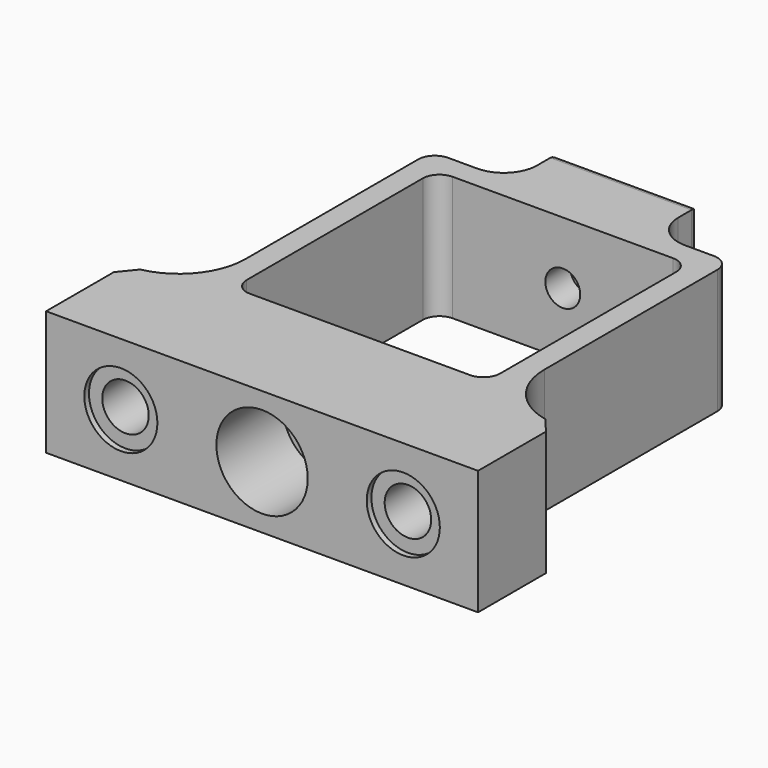
from build123d import *

# Parameters (mm, degrees)
F1_DEPTH       = 15
F2_T1_DEPTH    = 24.3030738828
F4_R           = 5.5
F5_DEPTH       = 6
F6_R           = 1
F7_R           = 2.1
F8_DEPTH       = 3.75
F9_R           = 5.5
F10_DEPTH      = 10
F10_DEPTH_BACK = 25
F11_R          = 2.1
F12_DEPTH      = 14.75
F3_R           = 2.8
F13_DEPTH      = 6.5
F14_R          = 4.4
F15_DEPTH      = 0.7


# Not quite as in the source:
# - a fillet or chamfer that OpenCascade refuses, or shapes differently, is made with other operations: its cross-section is extruded or revolved along the edge and cut away or added


with BuildPart() as f1:
    # F0 (on Top) → F1 (new body)
    with BuildSketch(Plane.XY):
        with BuildLine():
            ThreePointArc((18, 16), (17.4142135624, 17.4142135624), (16, 18))
            Line((16, 18), (12.5, 18))
            ThreePointArc((12.5, 18), (9.6715728753, 19.1715728753), (8.5, 22))
            Line((8.5, 22), (8.5, 25))
            Line((8.5, 25), (-8.5, 25))
            Line((-8.5, 25), (-8.5, 22))
            ThreePointArc((-8.5, 22), (-9.6715728753, 19.1715728753), (-12.5, 18))
            Line((-12.5, 18), (-16, 18))
            ThreePointArc((-16, 18), (-17.4142135624, 17.4142135624), (-18, 16))
            Line((-18, 16), (-18, -10))
            ThreePointArc((-18, -10), (-20.3431457505, -15.6568542495), (-26, -18))
            Line((-26, -18), (-26, -30))
            Line((-26, -30), (26, -30))
            Line((26, -30), (26, -18))
            ThreePointArc((26, -18), (20.3431457505, -15.6568542495), (18, -10))
            Line((18, -10), (18, 16))
        make_face()
        with BuildLine():
            Line((-13.25, 15.25), (13.25, 15.25))
            ThreePointArc((13.25, 15.25), (14.6642135624, 14.6642135624), (15.25, 13.25))
            Line((15.25, 13.25), (15.25, -13.25))
            ThreePointArc((15.25, -13.25), (14.6642135624, -14.6642135624), (13.25, -15.25))
            Line((13.25, -15.25), (-13.25, -15.25))
            ThreePointArc((-13.25, -15.25), (-14.6642135624, -14.6642135624), (-15.25, -13.25))
            Line((-15.25, -13.25), (-15.25, 13.25))
            ThreePointArc((-15.25, 13.25), (-14.6642135624, 14.6642135624), (-13.25, 15.25))
        make_face(mode=Mode.SUBTRACT)
    extrude(amount=F1_DEPTH)

    # F2: chamfer of 2 on 2 edges, made by hand

    # F2_s2 → F2_t1 (cut)
    with BuildSketch(Plane.XY.offset(-4.6515369414)):
        with BuildLine():
            Line((-24.4, -17.8383671769), (-26, -19.7979589711))
            Line((-26, -19.7979589711), (-26, -18))
            ThreePointArc((-26, -18), (-25.1675484588, -17.9565711479), (-24.4, -17.8383671769))
        make_face()
        with BuildLine():
            Line((26, -19.7979589711), (24.4, -17.8383671769))
            ThreePointArc((24.4, -17.8383671769), (25.1675484588, -17.9565711479), (26, -18))
            Line((26, -18), (26, -19.7979589711))
        make_face()
    extrude(amount=F2_T1_DEPTH, mode=Mode.SUBTRACT)

    # F4 (on face) → F5 (cut)
    with BuildSketch(Plane(origin=(0, 25, 0), x_dir=(-1, 0, 0), z_dir=(0, 1, 0))):
        with Locations((0, 7.5)):
            Circle(F4_R)
    extrude(amount=-F5_DEPTH, mode=Mode.SUBTRACT)

    # F6
    f6_edges = [f1.edges().sort_by_distance(p)[0] for p in [
        (0, 25, 0),
        (-8.5, 25, 7.5),
        (0, 25, 15),
        (8.5, 25, 7.5),
    ]]
    fillet(f6_edges, radius=F6_R)

    # F7 (on face) → F8 (cut, through all)
    with BuildSketch(Plane(origin=(0, 19, 0), x_dir=(-1, 0, 0), z_dir=(0, 1, 0))):
        with Locations((0, 7.5)):
            Circle(F7_R)
    extrude(amount=-F8_DEPTH, mode=Mode.SUBTRACT)

    # F9 (on face) → F10 (cut, two sides)
    with BuildSketch(Plane.XZ.offset(30)) as f10_sk:
        with Locations((0, 7.5)):
            Circle(F9_R)
    extrude(amount=-F10_DEPTH, mode=Mode.SUBTRACT)
    extrude(f10_sk.sketch, amount=F10_DEPTH_BACK, mode=Mode.SUBTRACT)

    # F11 (on face) → F12 (cut, through all)
    with BuildSketch(Plane.XZ.offset(30)):
        with Locations((0, 7.5)):
            Circle(F11_R)
    extrude(amount=-F12_DEPTH, mode=Mode.SUBTRACT)

    # F3 (on face) → F13 (cut)
    with BuildSketch(Plane.XZ.offset(30)):
        with Locations((-17, 7.5)):
            Circle(F3_R)
        with Locations((17, 7.5)):
            Circle(F3_R)
    extrude(amount=-F13_DEPTH, mode=Mode.SUBTRACT)

    # F14 (on face) → F15 (cut)
    with BuildSketch(Plane.XZ.offset(30)):
        with Locations((17, 7.5)):
            Circle(F14_R)
        with Locations((-17, 7.5)):
            Circle(F14_R)
    extrude(amount=-F15_DEPTH, mode=Mode.SUBTRACT)


solid = f1.part
